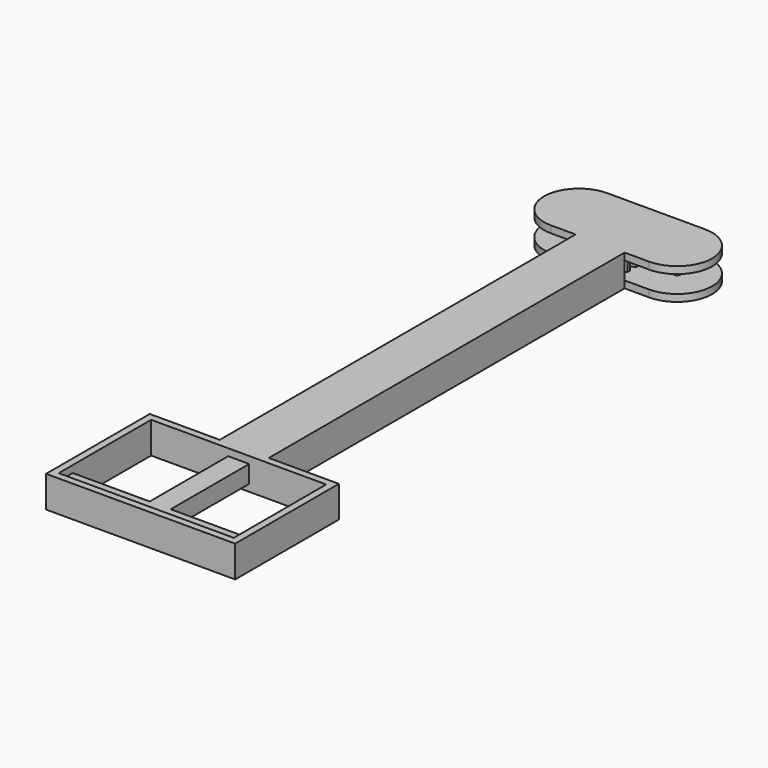
from build123d import *

# Parameters (mm, degrees)
F1_DEPTH      = 5
F3_W          = 50
F3_H          = 5
F4_DEPTH      = 5
F5_W          = 50
F5_H          = 33
F6_DEPTH      = 7
F6_DEPTH_BACK = 2
F9_DEPTH      = 5
F10_W         = 10
F10_H         = 5
F11_DEPTH     = 50
F12_R         = 1
F13_DEPTH     = 5


with BuildPart() as f1:
    # F0 (on Top) → F1 (new body)
    with BuildSketch(Plane.XY):
        Polygon((3, 11.0871235167), (3, 13), (0, 13), (0, -167), (3, -167), (3, -39.0871235167), (3, -36.9128764833), (3, -35.8871235167), (3, -33.7128764833), (3, -32.6871235167), (3, -30.5128764833), (3, -29.4871235167), (3, -27.3128764833), (3, -26.2871235167), (3, -24.1128764833), (3, -23.0871235167), (3, -20.9128764833), (3, -19.8871235167), (3, -17.7128764833), (3, -16.6871235167), (3, -14.5128764833), (3, -13.4871235167), (3, -11.3128764833), (3, -10.2871235167), (3, -8.1128764833), (3, -7.0871235167), (3, -4.9128764833), (3, -3.8871235167), (3, -1.7128764833), (3, -0.6871235167), (3, 1.4871235167), (3, 2.5128764833), (3, 4.6871235167), (3, 5.7128764833), (3, 7.8871235167), (3, 8.9128764833), align=None)
        with BuildLine():
            ThreePointArc((5, 10.5), (4.0421988802, 10.9373096378), (3, 11.0871235167))
            Line((3, 11.0871235167), (3, 8.9128764833))
            ThreePointArc((3, 8.9128764833), (4.0421988802, 9.0626903622), (5, 9.5))
            Line((5, 9.5), (5, 10))
            Line((5, 10), (5, 10.5))
        make_face()
        with BuildLine():
            ThreePointArc((5, 7.3), (4.0421988802, 7.7373096378), (3, 7.8871235167))
            Line((3, 7.8871235167), (3, 5.7128764833))
            ThreePointArc((3, 5.7128764833), (4.0421988802, 5.8626903622), (5, 6.3))
            Line((5, 6.3), (5, 6.8))
            Line((5, 6.8), (5, 7.3))
        make_face()
        with BuildLine():
            Line((3, -36.9128764833), (3, -39.0871235167))
            ThreePointArc((3, -39.0871235167), (4.0421988802, -38.9373096378), (5, -38.5))
            Line((5, -38.5), (5, -38))
            Line((5, -38), (5, -37.5))
            ThreePointArc((5, -37.5), (4.0421988802, -37.0626903622), (3, -36.9128764833))
        make_face()
        with BuildLine():
            ThreePointArc((5, 4.1), (4.0421988802, 4.5373096378), (3, 4.6871235167))
            Line((3, 4.6871235167), (3, 2.5128764833))
            ThreePointArc((3, 2.5128764833), (4.0421988802, 2.6626903622), (5, 3.1))
            Line((5, 3.1), (5, 3.6))
            Line((5, 3.6), (5, 4.1))
        make_face()
        with BuildLine():
            Line((3, -33.7128764833), (3, -35.8871235167))
            ThreePointArc((3, -35.8871235167), (4.0421988802, -35.7373096378), (5, -35.3))
            Line((5, -35.3), (5, -34.8))
            Line((5, -34.8), (5, -34.3))
            ThreePointArc((5, -34.3), (4.0421988802, -33.8626903622), (3, -33.7128764833))
        make_face()
        with BuildLine():
            ThreePointArc((5, 0.9), (4.0421988802, 1.3373096378), (3, 1.4871235167))
            Line((3, 1.4871235167), (3, -0.6871235167))
            ThreePointArc((3, -0.6871235167), (4.0421988802, -0.5373096378), (5, -0.1))
            Line((5, -0.1), (5, 0.4))
            Line((5, 0.4), (5, 0.9))
        make_face()
        with BuildLine():
            Line((3, -30.5128764833), (3, -32.6871235167))
            ThreePointArc((3, -32.6871235167), (4.0421988802, -32.5373096378), (5, -32.1))
            Line((5, -32.1), (5, -31.6))
            Line((5, -31.6), (5, -31.1))
            ThreePointArc((5, -31.1), (4.0421988802, -30.6626903622), (3, -30.5128764833))
        make_face()
        with BuildLine():
            ThreePointArc((5, -2.3), (4.0421988802, -1.8626903622), (3, -1.7128764833))
            Line((3, -1.7128764833), (3, -3.8871235167))
            ThreePointArc((3, -3.8871235167), (4.0421988802, -3.7373096378), (5, -3.3))
            Line((5, -3.3), (5, -2.8))
            Line((5, -2.8), (5, -2.3))
        make_face()
        with BuildLine():
            Line((3, -27.3128764833), (3, -29.4871235167))
            ThreePointArc((3, -29.4871235167), (4.0421988802, -29.3373096378), (5, -28.9))
            Line((5, -28.9), (5, -28.4))
            Line((5, -28.4), (5, -27.9))
            ThreePointArc((5, -27.9), (4.0421988802, -27.4626903622), (3, -27.3128764833))
        make_face()
        with BuildLine():
            ThreePointArc((5, -5.5), (4.0421988802, -5.0626903622), (3, -4.9128764833))
            Line((3, -4.9128764833), (3, -7.0871235167))
            ThreePointArc((3, -7.0871235167), (4.0421988802, -6.9373096378), (5, -6.5))
            Line((5, -6.5), (5, -6))
            Line((5, -6), (5, -5.5))
        make_face()
        with BuildLine():
            Line((3, -24.1128764833), (3, -26.2871235167))
            ThreePointArc((3, -26.2871235167), (4.0421988802, -26.1373096378), (5, -25.7))
            Line((5, -25.7), (5, -25.2))
            Line((5, -25.2), (5, -24.7))
            ThreePointArc((5, -24.7), (4.0421988802, -24.2626903622), (3, -24.1128764833))
        make_face()
        with BuildLine():
            ThreePointArc((5, -8.7), (4.0421988802, -8.2626903622), (3, -8.1128764833))
            Line((3, -8.1128764833), (3, -10.2871235167))
            ThreePointArc((3, -10.2871235167), (4.0421988802, -10.1373096378), (5, -9.7))
            Line((5, -9.7), (5, -9.2))
            Line((5, -9.2), (5, -8.7))
        make_face()
        with BuildLine():
            Line((3, -20.9128764833), (3, -23.0871235167))
            ThreePointArc((3, -23.0871235167), (4.0421988802, -22.9373096378), (5, -22.5))
            Line((5, -22.5), (5, -22))
            Line((5, -22), (5, -21.5))
            ThreePointArc((5, -21.5), (4.0421988802, -21.0626903622), (3, -20.9128764833))
        make_face()
        with BuildLine():
            ThreePointArc((5, -11.9), (4.0421988802, -11.4626903622), (3, -11.3128764833))
            Line((3, -11.3128764833), (3, -13.4871235167))
            ThreePointArc((3, -13.4871235167), (4.0421988802, -13.3373096378), (5, -12.9))
            Line((5, -12.9), (5, -12.4))
            Line((5, -12.4), (5, -11.9))
        make_face()
        with BuildLine():
            Line((3, -17.7128764833), (3, -19.8871235167))
            ThreePointArc((3, -19.8871235167), (4.0421988802, -19.7373096378), (5, -19.3))
            Line((5, -19.3), (5, -18.8))
            Line((5, -18.8), (5, -18.3))
            ThreePointArc((5, -18.3), (4.0421988802, -17.8626903622), (3, -17.7128764833))
        make_face()
        with BuildLine():
            ThreePointArc((5, -15.1), (4.0421988802, -14.6626903622), (3, -14.5128764833))
            Line((3, -14.5128764833), (3, -16.6871235167))
            ThreePointArc((3, -16.6871235167), (4.0421988802, -16.5373096378), (5, -16.1))
            Line((5, -16.1), (5, -15.6))
            Line((5, -15.6), (5, -15.1))
        make_face()
    extrude(amount=F1_DEPTH)

    # F2: F1 across face


with BuildPart() as f1_1:
    add(f1.part)
    add(f1.part.mirror(Plane(origin=(0, -77, 2.5), x_dir=(0, -1, 0), z_dir=(-1, 0, 0))))

    # F3 (on face) → F4 (join)
    with BuildSketch(Plane.XZ.offset(167)):
        with Locations((0, 2.5)):
            Rectangle(F3_W, F3_H)
    extrude(amount=F4_DEPTH)


with BuildPart() as f6:
    # F5 (on Top) → F6 (new body, two sides)
    with BuildSketch(Plane.XY) as f6_sk:
        with BuildLine():
            ThreePointArc((14, -10), (21.0710678119, -7.0710678119), (24, 0))
            ThreePointArc((24, 0), (21.0710678119, 7.0710678119), (14, 10))
            ThreePointArc((14, 10), (4, 0), (14, -10))
        make_face()
        with BuildLine():
            ThreePointArc((14, -10), (4, 0), (14, 10))
            Line((14, 10), (0, 10))
            Line((0, 10), (-14, 10))
            ThreePointArc((-14, 10), (-6.9289321881, 7.0710678119), (-4, 0))
            ThreePointArc((-4, 0), (-6.9289321881, -7.0710678119), (-14, -10))
            Line((-14, -10), (-7, -10))
            Line((-7, -10), (-7, -137))
            Line((-7, -137), (-27, -137))
            Line((-27, -137), (-27, -174))
            Line((-27, -174), (0, -174))
            Line((0, -174), (27, -174))
            Line((27, -174), (27, -137))
            Line((27, -137), (7, -137))
            Line((7, -137), (7, -10))
            Line((7, -10), (14, -10))
        make_face()
        with Locations((0, -155.5)):
            Rectangle(F5_W, F5_H, mode=Mode.SUBTRACT)
        with BuildLine():
            ThreePointArc((-4, 0), (-6.9289321881, 7.0710678119), (-14, 10))
            ThreePointArc((-14, 10), (-24, 0), (-14, -10))
            ThreePointArc((-14, -10), (-6.9289321881, -7.0710678119), (-4, 0))
        make_face()
    extrude(amount=F6_DEPTH)
    extrude(f6_sk.sketch, amount=-F6_DEPTH_BACK)

    # F7: cut F1
    add(f1_1.part, mode=Mode.SUBTRACT)

    # F8 (on Top) → F9 (cut)
    with BuildSketch(Plane.XY):
        with BuildLine():
            ThreePointArc((-14, 10), (-24, 0), (-14, -10))
            Line((-14, -10), (14, -10))
            ThreePointArc((14, -10), (24, 0), (14, 10))
            Line((14, 10), (-14, 10))
        make_face()
    extrude(amount=F9_DEPTH, mode=Mode.SUBTRACT)

    # F10 (on face) → F11 (cut)
    with BuildSketch(Plane(origin=(0, -10, 0), x_dir=(-1, 0, 0), z_dir=(0, 1, 0))):
        with Locations((0, 2.5)):
            Rectangle(F10_W, F10_H)
    extrude(amount=-F11_DEPTH, mode=Mode.SUBTRACT)

    # F12 (on Top) → F13 (join, through all)
    with BuildSketch(Plane.XY):
        with Locations((-14, 0)):
            Circle(F12_R)
        with Locations((14, 0)):
            Circle(F12_R)
    extrude(amount=F13_DEPTH)


solid = Compound([f1_1.part, f6.part])
